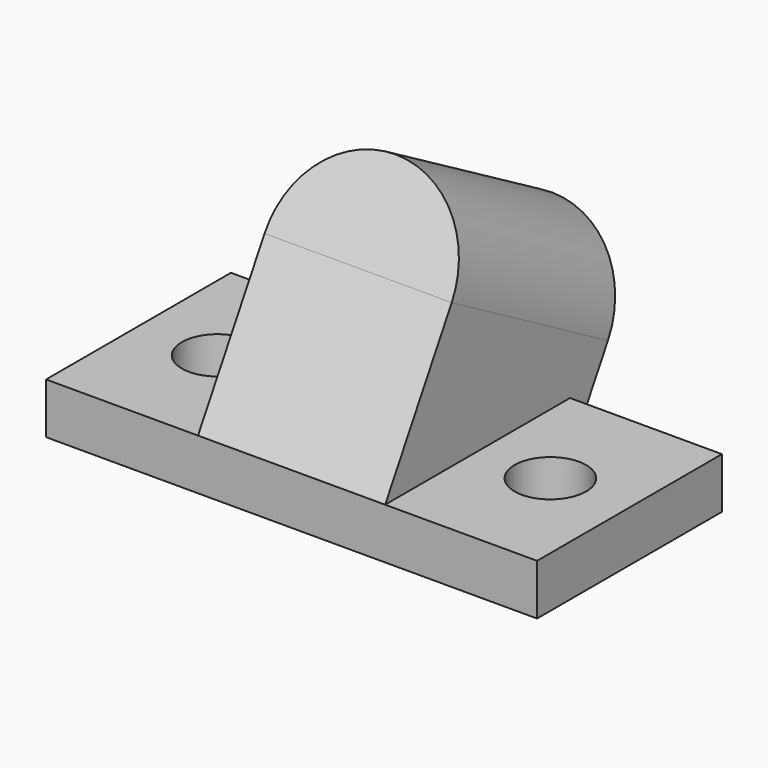
from build123d import *

# Parameters (mm, degrees)
F0_W     = 107.95
F0_H     = 50.8
F0_R     = 7.874
F1_DEPTH = 11.176
F3_DEPTH = 33.401
F4_DEPTH = 41.148
F5_DEPTH = 33.401
F6_W     = 41.148
F6_H     = 20.574
F7_DEPTH = 49.5820905122
F8_R     = 20.57399


# Not quite as in the source:
# - a fillet or chamfer is up to 0.001 mm smaller than in the source, because OpenCascade refuses the exact size


with BuildPart() as f1:
    # F0 (on Top) → F1 (new body)
    with BuildSketch(Plane.XY):
        with Locations((18.2708286419, 0.7708109915)):
            Rectangle(F0_W, F0_H)
        with Locations((-18.3051713581, 0.7708109915)):
            Circle(F0_R, mode=Mode.SUBTRACT)
        with Locations((54.8468286419, 0.7708109915)):
            Circle(F0_R, mode=Mode.SUBTRACT)
    extrude(amount=F1_DEPTH)



with BuildPart() as f3:
    # F2 (on face) → F3 (new body)
    with BuildSketch(Plane(origin=(-35.7041713581, 0, 0), x_dir=(0, -1, 0), z_dir=(-1, 0, 0))):
        Polygon((-26.1708109915, 11.176), (24.6291890085, 11.176), (6.3411890085, 42.8517451688), (-36.5981609479, 18.0606999127), (-26.1708109915, 0), align=None)
    extrude(amount=-F3_DEPTH)


with BuildPart() as f1_1:
    add(f1.part)
    # F4 (add): a face of the model
    f4_faces = [f3.part.faces().sort_by_distance(p)[0] for p in [
        (-2.3031713581, 4.9580328492, 21.6795412193),
    ]]

    add(f3.part)  # F4 merges F3
    extrude(f4_faces, amount=F4_DEPTH)

    # F2 (on face) → F5 (cut)
    with BuildSketch(Plane(origin=(-35.7041713581, 0, 0), x_dir=(0, -1, 0), z_dir=(-1, 0, 0))):
        Polygon((-26.1708109915, 11.176), (24.6291890085, 11.176), (6.3411890085, 42.8517451688), (-36.5981609479, 18.0606999127), (-26.1708109915, 0), align=None)
    extrude(amount=-F5_DEPTH, mode=Mode.SUBTRACT)

    # F6 (on face) → F7 (join, through all)
    with BuildSketch(Plane(origin=(0, -23.3112417127, 13.458751678), x_dir=(1, 0, 0), z_dir=(0, -0.8660254038, 0.5))):
        with Locations((18.2708286419, 44.2271054085)):
            Rectangle(F6_W, F6_H)
    extrude(amount=-F7_DEPTH)

    # F8 (radius 20.574 in the source; OpenCascade refuses exactly that, so slightly less here)
    f8_edges = [f1_1.edges().sort_by_distance(p)[0] for p in [
        (38.844829, 25.415486, 48.273829),
        (-2.303171, 25.415486, 48.273829),
    ]]
    fillet(f8_edges, radius=F8_R)


solid = f1_1.part
